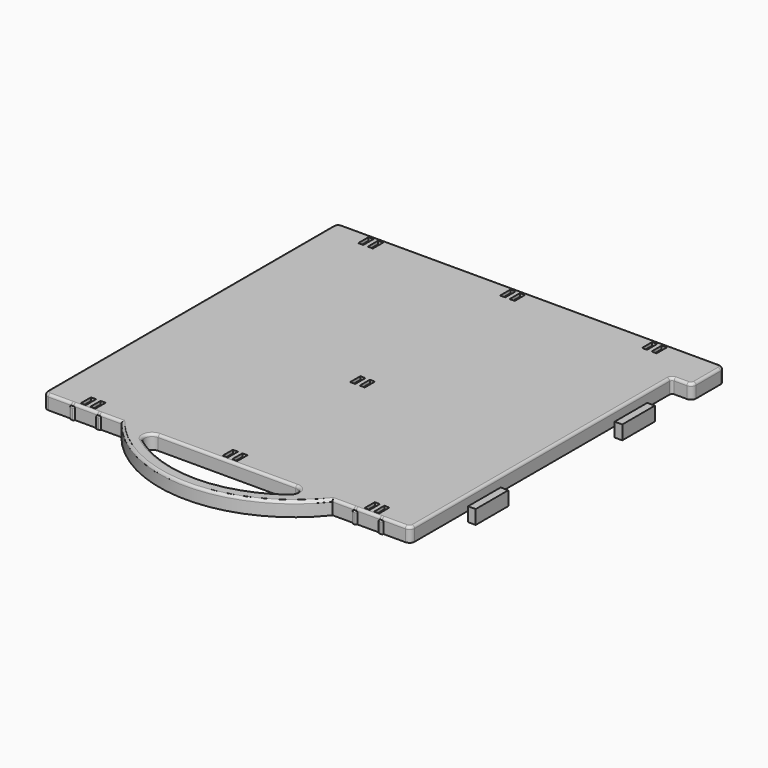
from build123d import *

# Parameters (mm, degrees)
F0_W      = 12.7
F0_H      = 25.4
F1_DEPTH  = 8.89
F2_R      = 3.175
F3_R      = 1.5875
F4_W      = 3.175
F4_H      = 7.9375
F5_DEPTH  = 8.891
F6_W      = 2.778125
F6_H      = 7.3421875
F7_DEPTH  = 0.79375
F8_R      = 0.79374
F9_W      = 25.4
F9_H      = 8.73125
F10_DEPTH = 4.7625
F11_W     = 25.4
F11_H     = 8.73125
F12_DEPTH = 4.7625
F14_DEPTH = 8.89
F15_R     = 4.7625
F16_R     = 1.5875
F18_DEPTH = 6.89


# Not quite as in the source:
# - a fillet or chamfer is up to 0.001 mm smaller than in the source, because OpenCascade refuses the exact size


with BuildPart() as f1:
    # F0 (on Top) → F1 (new body)
    with BuildSketch(Plane.XY):
        Polygon((114.4984375, 89.0984375), (114.4984375, 114.4984375), (-114.4984375, 114.4984375), (-114.4984375, -114.4984375), (114.4984375, -114.4984375), align=None)
        with Locations((120.8484375, 101.7984375)):
            Rectangle(F0_W, F0_H)
    extrude(amount=F1_DEPTH)

    # F2
    f2_edges = [f1.edges().sort_by_distance(p)[0] for p in [
        (127.198438, 114.498438, 4.445),
        (127.198438, 89.098438, 4.445),
        (-114.498437, 114.498437, 4.445),
        (-114.498438, -114.498437, 4.445),
        (114.498438, -114.498437, 4.445),
    ]]
    fillet(f2_edges, radius=F2_R)

    # F3
    f3_edges = [f1.edges().sort_by_distance(p)[0] for p in [
        (114.498438, 89.098438, 4.445),
    ]]
    fillet(f3_edges, radius=F3_R)

    # F4 (on face) → F5 (cut, through all)
    with BuildSketch(Plane.XY.offset(8.89)):
        Polygon((-1.3890625, 104.1796875), (-1.3890625, 112.1171875), (-4.5640625, 112.1171875), (-4.5640625, 104.1796875), align=None)
        with Locations((-85.5265625, 108.1484375)):
            Rectangle(F4_W, F4_H)
        with Locations((-91.4796875, 108.1484375)):
            Rectangle(F4_W, F4_H)
        Polygon((87.1140625, 112.1171875), (83.9390625, 112.1171875), (83.9390625, 104.1796875), (87.1140625, 104.1796875), align=None)
        Polygon((4.5640625, 112.1171875), (1.3890625, 112.1171875), (1.3890625, 104.1796875), (4.5640625, 104.1796875), align=None)
        with Locations((91.4796875, 108.1484375)):
            Rectangle(F4_W, F4_H)
        Polygon((-1.3890625, -112.1171875), (-1.3890625, -104.1796875), (-4.5640625, -104.1796875), (-4.5640625, -112.1171875), align=None)
        with Locations((-85.5265625, -108.1484375)):
            Rectangle(F4_W, F4_H)
        Polygon((4.5640625, -104.1796875), (1.3890625, -104.1796875), (1.3890625, -112.1171875), (4.5640625, -112.1171875), align=None)
        with Locations((-91.4796875, -108.1484375)):
            Rectangle(F4_W, F4_H)
        Polygon((83.9390625, -104.1796875), (83.9390625, -112.1171875), (87.1140625, -112.1171875), (87.1140625, -104.1796875), align=None)
        Polygon((93.0671875, -104.1796875), (89.8921875, -104.1796875), (89.8921875, -112.1171875), (93.0671875, -112.1171875), align=None)
        Polygon((-1.3890625, -12.7396875), (-1.3890625, -4.8021875), (-4.5640625, -4.8021875), (-4.5640625, -12.7396875), align=None)
        with Locations((2.9765625, -8.7709375)):
            Rectangle(F4_W, F4_H)
    extrude(amount=-F5_DEPTH, mode=Mode.SUBTRACT)

    # F6 (on face) → F7 (join)
    with BuildSketch(Plane.XZ.offset(114.4984375)):
        with Locations((-96.2421875, 3.67109375)):
            Rectangle(F6_W, F6_H)
        with Locations((-79.9703125, 3.67109375)):
            Rectangle(F6_W, F6_H)
        with Locations((96.2421875, 3.67109375)):
            Rectangle(F6_W, F6_H)
        with Locations((79.9703125, 3.67109375)):
            Rectangle(F6_W, F6_H)
    extrude(amount=F7_DEPTH)

    # F8 (radius 0.79375 in the source; OpenCascade refuses exactly that, so slightly less here)
    f8_edges = [f1.edges().sort_by_distance(p)[0] for p in [
        (78.58125, -115.292187, 3.671094),
        (81.359375, -115.292187, 3.671094),
        (81.359375, -114.895312, 7.342188),
        (78.58125, -114.895312, 7.342188),
        (79.970313, -115.292187, 7.342188),
        (97.63125, -114.895312, 7.342188),
        (94.853125, -114.895312, 7.342188),
        (96.242188, -115.292187, 7.342188),
        (97.63125, -115.292187, 3.671094),
        (94.853125, -115.292187, 3.671094),
        (-97.63125, -114.895312, 7.342187),
        (-94.853125, -114.895312, 7.342187),
        (-81.359375, -114.895312, 7.342188),
        (-78.58125, -114.895312, 7.342188),
        (-79.970313, -115.292187, 7.342188),
        (-96.242188, -115.292187, 7.342188),
        (-97.63125, -115.292187, 3.671094),
        (-81.359375, -115.292187, 3.671094),
        (-78.58125, -115.292187, 3.671094),
        (-94.853125, -115.292187, 3.671094),
    ]]
    fillet(f8_edges, radius=F8_R)

    # F9 (on face) → F10 (join)
    with BuildSketch(Plane.YZ.offset(114.4984375)):
        with Locations((57.3484375, -1.825625)):
            Rectangle(F9_W, F9_H)
        with Locations((-56.9515625, -1.825625)):
            Rectangle(F9_W, F9_H)
    extrude(amount=F10_DEPTH)

    # F11 (on face) → F12 (join)
    with BuildSketch(Plane(origin=(-114.4984375, 0, 0), x_dir=(0, -1, 0), z_dir=(-1, 0, 0))):
        with Locations((-57.3484375, -1.825625)):
            Rectangle(F11_W, F11_H)
        with Locations((56.9515625, -1.825625)):
            Rectangle(F11_W, F11_H)
    extrude(amount=F12_DEPTH)

    # F13 (on face) → F14 (join, through all)
    with BuildSketch(Plane.XY.offset(8.89)):
        with BuildLine():
            Line((-55.373663482, -114.4984375), (-65.88125, -114.4984375))
            ThreePointArc((-65.88125, -114.4984375), (-36.5663835656, -137.8968862902), (-2.027e-07, -146.2484375))
            ThreePointArc((-2.027e-07, -146.2484375), (36.566383383, -137.8968863782), (65.88125, -114.4984375))
            Line((65.88125, -114.4984375), (55.373663482, -114.4984375))
            ThreePointArc((55.373663482, -114.4984375), (30.1383383901, -132.1054288842), (0, -138.3109375))
            ThreePointArc((0, -138.3109375), (-30.1383383901, -132.1054288842), (-55.373663482, -114.4984375))
        make_face()
    extrude(amount=-F14_DEPTH)

    # F15
    f15_edges = [f1.edges().sort_by_distance(p)[0] for p in [
        (-55.373663, -114.498437, 4.445),
        (55.373663, -114.498437, 4.445),
    ]]
    fillet(f15_edges, radius=F15_R)

    # F16
    f16_edges = [f1.edges().sort_by_distance(p)[0] for p in [
        (0, -138.310938, 8.89),
        (88.602344, -114.498437, 8.89),
        (0, -146.248438, 8.89),
    ]]
    fillet(f16_edges, radius=F16_R)

    # F17 (on face) → F18 (cut, through all)
    with BuildSketch(Plane(origin=(0, 0, 0), x_dir=(1, 0, 0), z_dir=(0, 0, -1))):
        with BuildLine():
            Line((111.3234375, 112.1484375), (-111.3234375, 112.1484375))
            ThreePointArc((-111.3234375, 112.1484375), (-111.9068005945, 111.9068005945), (-112.1484375, 111.3234375))
            Line((-112.1484375, 111.3234375), (-112.1484375, 44.2515625))
            Line((-112.1484375, 44.2515625), (-112.1484375, -44.6484375))
            Line((-112.1484375, -44.6484375), (-112.1484375, -111.3234375))
            ThreePointArc((-112.1484375, -111.3234375), (-111.9068005945, -111.9068005945), (-111.3234375, -112.1484375))
            Line((-111.3234375, -112.1484375), (120.662458241, -112.1484375))
            Line((120.662458241, -112.1484375), (124.0234375, -112.1484375))
            ThreePointArc((124.0234375, -112.1484375), (124.6068005945, -111.9068005945), (124.8484375, -111.3234375))
            Line((124.8484375, -111.3234375), (124.8484375, -92.2734375))
            ThreePointArc((124.8484375, -92.2734375), (124.6068005945, -91.6900744055), (124.0234375, -91.4484375))
            Line((124.0234375, -91.4484375), (116.0859375, -91.4484375))
            ThreePointArc((116.0859375, -91.4484375), (113.3017045491, -90.2951704509), (112.1484375, -87.5109375))
            Line((112.1484375, -87.5109375), (112.1484375, 111.3234375))
            ThreePointArc((112.1484375, 111.3234375), (111.9068005945, 111.9068005945), (111.3234375, 112.1484375))
        make_face()
    extrude(amount=-F18_DEPTH, mode=Mode.SUBTRACT)


solid = f1.part
